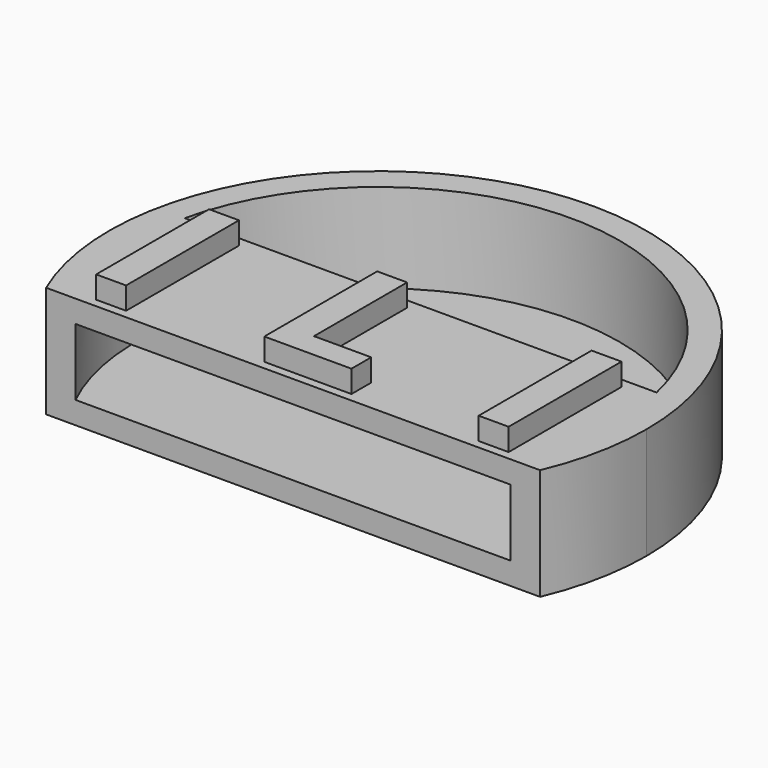
from build123d import *

# Parameters (mm, degrees)
F0_W         = 1.3418249954
F0_H         = 6.3269333375
F1_DEPTH     = 5
F0_TEXT_SIZE = 8.8624148304
F2_DEPTH     = 6
F3_DEPTH     = 4
F4_DEPTH     = 1


# Not quite as in the source:
# - a feature names something its author has since deleted; it is built from what else it names
# - Text() gives the source's letters only with a copy of the font that has no kerning and outlines rounded to 1/6400 em; it was checked with that copy


with BuildPart() as f1:
    # F0 (on Top) → F1 (new body)
    with BuildSketch(Plane.XY):
        with BuildLine():
            ThreePointArc((-10.5812333875, 2.4), (-10.7782748651, -1.2455083027), (-9.7549987186, -4.75))
            Line((-9.7549987186, -4.75), (9.7549987186, -4.75))
            ThreePointArc((9.7549987186, -4.75), (10.5727062784, -2.4372898784), (10.85, 0))
            ThreePointArc((10.85, 0), (10.7825989969, 1.2075010861), (10.5812333875, 2.4))
            Line((10.5812333875, 2.4), (0, 2.4))
            Line((0, 2.4), (-10.5812333875, 2.4))
        make_face()
        with Locations((-8.4656832915, -1.2024720091)):
            Rectangle(F0_W, F0_H, mode=Mode.SUBTRACT)
        Polygon((2.3111516175, -4.3659386779), (-1.5966194218, -4.3659386779), (-1.5966194218, 1.9609946596), (-0.2547944264, 1.9609946596), (-0.2547944264, -3.2581368241), (2.3111516175, -3.2581368241), align=None, mode=Mode.SUBTRACT)
        with Locations((8.6872436623, -1.2024720091)):
            Rectangle(F0_W, F0_H, mode=Mode.SUBTRACT)
        with BuildLine():
            ThreePointArc((11.0742945599, -4.75), (11.8035534787, -2.4245876508), (12.05, 0))
            ThreePointArc((12.05, 0), (-2.4245876508, 11.8035534787), (-11.0742945599, -4.75))
            Line((-11.0742945599, -4.75), (-9.7549987186, -4.75))
            ThreePointArc((-9.7549987186, -4.75), (-10.7782748651, -1.2455083027), (-10.5812333875, 2.4))
            ThreePointArc((-10.5812333875, 2.4), (0, 10.85), (10.5812333875, 2.4))
            ThreePointArc((10.5812333875, 2.4), (10.7825989969, 1.2075010861), (10.85, 0))
            ThreePointArc((10.85, 0), (10.5727062784, -2.4372898784), (9.7549987186, -4.75))
            Line((9.7549987186, -4.75), (11.0742945599, -4.75))
        make_face()
    extrude(amount=F1_DEPTH)

    # F0 (on Top) → F2 (join)
    with BuildSketch(Plane.XY):
        with Locations((-9.9328283717, -4.3659386779)):
            Text('I  L  I', F0_TEXT_SIZE, font='Open Sans', font_style=FontStyle.BOLD, text_align=(TextAlign.LEFT, TextAlign.BOTTOM))
    extrude(amount=F2_DEPTH)

    # F0 (on Top) → F3 (cut)
    with BuildSketch(Plane.XY):
        with BuildLine():
            ThreePointArc((-10.5812333875, 2.4), (-10.7782748651, -1.2455083027), (-9.7549987186, -4.75))
            Line((-9.7549987186, -4.75), (9.7549987186, -4.75))
            ThreePointArc((9.7549987186, -4.75), (10.5727062784, -2.4372898784), (10.85, 0))
            ThreePointArc((10.85, 0), (10.7825989969, 1.2075010861), (10.5812333875, 2.4))
            Line((10.5812333875, 2.4), (0, 2.4))
            Line((0, 2.4), (-10.5812333875, 2.4))
        make_face()
        with Locations((-8.4656832915, -1.2024720091)):
            Rectangle(F0_W, F0_H, mode=Mode.SUBTRACT)
        Polygon((2.3111516175, -4.3659386779), (-1.5966194218, -4.3659386779), (-1.5966194218, 1.9609946596), (-0.2547944264, 1.9609946596), (-0.2547944264, -3.2581368241), (2.3111516175, -3.2581368241), align=None, mode=Mode.SUBTRACT)
        with Locations((8.6872436623, -1.2024720091)):
            Rectangle(F0_W, F0_H, mode=Mode.SUBTRACT)
        with Locations((-9.9328283717, -4.3659386779)):
            Text('I  L  I', F0_TEXT_SIZE, font='Open Sans', font_style=FontStyle.BOLD, text_align=(TextAlign.LEFT, TextAlign.BOTTOM))
    extrude(amount=F3_DEPTH, mode=Mode.SUBTRACT)

    # F0 (on Top) → F4 (join)
    with BuildSketch(Plane.XY):
        with BuildLine():
            ThreePointArc((10.5812333875, 2.4), (0, 10.85), (-10.5812333875, 2.4))
            Line((-10.5812333875, 2.4), (0, 2.4))
            Line((0, 2.4), (10.5812333875, 2.4))
        make_face()
        with BuildLine():
            ThreePointArc((2.35, 4.75), (1.6617009358, 3.0882990642), (0, 2.4))
            ThreePointArc((0, 2.4), (-1.6617009358, 6.4117009358), (2.35, 4.75))
        make_face(mode=Mode.SUBTRACT)
        with BuildLine():
            ThreePointArc((-10.5812333875, 2.4), (-10.7782748651, -1.2455083027), (-9.7549987186, -4.75))
            Line((-9.7549987186, -4.75), (9.7549987186, -4.75))
            ThreePointArc((9.7549987186, -4.75), (10.5727062784, -2.4372898784), (10.85, 0))
            ThreePointArc((10.85, 0), (10.7825989969, 1.2075010861), (10.5812333875, 2.4))
            Line((10.5812333875, 2.4), (0, 2.4))
            Line((0, 2.4), (-10.5812333875, 2.4))
        make_face()
        with Locations((-8.4656832915, -1.2024720091)):
            Rectangle(F0_W, F0_H, mode=Mode.SUBTRACT)
        Polygon((2.3111516175, -4.3659386779), (-1.5966194218, -4.3659386779), (-1.5966194218, 1.9609946596), (-0.2547944264, 1.9609946596), (-0.2547944264, -3.2581368241), (2.3111516175, -3.2581368241), align=None, mode=Mode.SUBTRACT)
        with Locations((8.6872436623, -1.2024720091)):
            Rectangle(F0_W, F0_H, mode=Mode.SUBTRACT)
        with Locations((-9.9328283717, -4.3659386779)):
            Text('I  L  I', F0_TEXT_SIZE, font='Open Sans', font_style=FontStyle.BOLD, text_align=(TextAlign.LEFT, TextAlign.BOTTOM))
    extrude(amount=F4_DEPTH)


solid = f1.part
